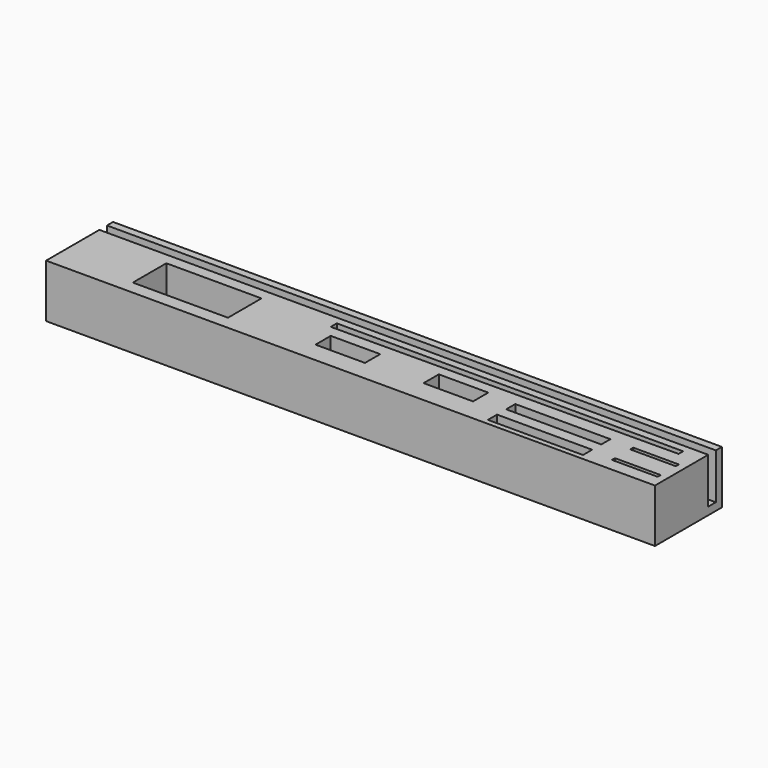
from build123d import *

# Parameters (mm, degrees)
F0_W     = 160
F0_H     = 17.5
F0_W_2   = 25
F0_H_2   = 11
F0_W_3   = 13
F0_H_3   = 5
F0_H_4   = 3
F0_W_4   = 12
F0_H_5   = 1
F0_H_6   = 2.5
F0_H_7   = 2
F1_DEPTH = 2
F2_DEPTH = 12
F3_DEPTH = 2
F4_DEPTH = 2


# Not quite as in the source:
# - a feature names something its author has since deleted; it is built from what else it names


with BuildPart() as f1:
    # F0 (on Top) → F1 (new body)
    with BuildSketch(Plane.XY):
        with Locations((-35.2099549949, 29.3164705649)):
            Rectangle(F0_W, F0_H)
        with Locations((-82.7099549949, 29.5664705649)):
            Rectangle(F0_W_2, F0_H_2, mode=Mode.SUBTRACT)
        with Locations((-42.2099549949, 28.443671599)):
            Rectangle(F0_W_3, F0_H_3, mode=Mode.SUBTRACT)
        with Locations((12.2900450051, 23.443671599)):
            Rectangle(F0_W_2, F0_H_4, mode=Mode.SUBTRACT)
        with Locations((36.7900450051, 24.443671599)):
            Rectangle(F0_W_4, F0_H_5, mode=Mode.SUBTRACT)
        with Locations((-14.2099549949, 28.943671599)):
            Rectangle(F0_W_3, F0_H_3, mode=Mode.SUBTRACT)
        with Locations((12.2900450051, 29.443671599)):
            Rectangle(F0_W_2, F0_H_4, mode=Mode.SUBTRACT)
        with Locations((36.7900450051, 30.443671599)):
            Rectangle(F0_W_4, F0_H_5, mode=Mode.SUBTRACT)
        Polygon((-51.2099549949, 36.0664705649), (39.7900450051, 36.0664705649), (39.7900450051, 34.5664705649), (-51.2099549949, 34.0664705649), align=None, mode=Mode.SUBTRACT)
        with Locations((-35.2099549949, 39.3164705649)):
            Rectangle(F0_W, F0_H_6)
        with Locations((-35.2099549949, 41.5664705649)):
            Rectangle(F0_W, F0_H_7)
        with Locations((-82.7099549949, 29.5664705649)):
            Rectangle(F0_W_2, F0_H_2)
        Polygon((39.7900450051, 34.5664705649), (39.7900450051, 36.0664705649), (-51.2099549949, 36.0664705649), (-51.2099549949, 34.0664705649), align=None)
        with Locations((12.2900450051, 23.443671599)):
            Rectangle(F0_W_2, F0_H_4)
        with Locations((-42.2099549949, 28.443671599)):
            Rectangle(F0_W_3, F0_H_3)
        with Locations((-14.2099549949, 28.943671599)):
            Rectangle(F0_W_3, F0_H_3)
        with Locations((36.7900450051, 24.443671599)):
            Rectangle(F0_W_4, F0_H_5)
        with Locations((36.7900450051, 30.443671599)):
            Rectangle(F0_W_4, F0_H_5)
    extrude(amount=-F1_DEPTH)

    # F0 (on Top) → F2 (join)
    with BuildSketch(Plane.XY):
        with Locations((-35.2099549949, 29.3164705649)):
            Rectangle(F0_W, F0_H)
        with Locations((-82.7099549949, 29.5664705649)):
            Rectangle(F0_W_2, F0_H_2, mode=Mode.SUBTRACT)
        with Locations((-42.2099549949, 28.443671599)):
            Rectangle(F0_W_3, F0_H_3, mode=Mode.SUBTRACT)
        with Locations((12.2900450051, 23.443671599)):
            Rectangle(F0_W_2, F0_H_4, mode=Mode.SUBTRACT)
        with Locations((36.7900450051, 24.443671599)):
            Rectangle(F0_W_4, F0_H_5, mode=Mode.SUBTRACT)
        with Locations((-14.2099549949, 28.943671599)):
            Rectangle(F0_W_3, F0_H_3, mode=Mode.SUBTRACT)
        with Locations((12.2900450051, 29.443671599)):
            Rectangle(F0_W_2, F0_H_4, mode=Mode.SUBTRACT)
        with Locations((36.7900450051, 30.443671599)):
            Rectangle(F0_W_4, F0_H_5, mode=Mode.SUBTRACT)
        Polygon((-51.2099549949, 36.0664705649), (39.7900450051, 36.0664705649), (39.7900450051, 34.5664705649), (-51.2099549949, 34.0664705649), align=None, mode=Mode.SUBTRACT)
        with Locations((-35.2099549949, 41.5664705649)):
            Rectangle(F0_W, F0_H_7)
    extrude(amount=F2_DEPTH)

    # F0 (on Top) → F3 (join)
    with BuildSketch(Plane.XY):
        with Locations((36.7900450051, 30.443671599)):
            Rectangle(F0_W_4, F0_H_5)
        with Locations((36.7900450051, 24.443671599)):
            Rectangle(F0_W_4, F0_H_5)
    extrude(amount=F3_DEPTH)

    # F0 (on Top) → F4 (join)
    with BuildSketch(Plane.XY):
        with Locations((12.2900450051, 29.443671599)):
            Rectangle(F0_W_2, F0_H_4)
    extrude(amount=F4_DEPTH)


solid = f1.part
